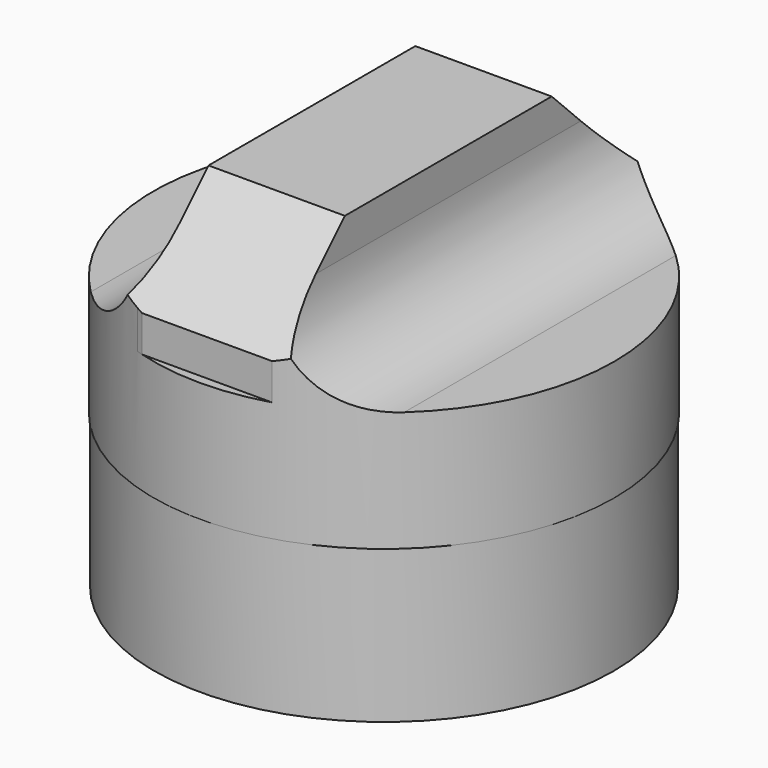
from build123d import *

# Parameters (mm, degrees)
F0_R         = 12.625
F0_R_2       = 10.375
F0_R_3       = 5
F1_DEPTH     = 15
F2_DEPTH     = 15
F3_R         = 12.6739646699
F4_DEPTH     = 6.6
F6_DEPTH     = 7
F7_T4_DEPTH  = 36.6039255786
F7_S5_R      = 12.6739646699
F7_T6_DEPTH  = 20
F7_T10_DEPTH = 24.210816556
F7_S11_R     = 12.6739646699
F7_T12_DEPTH = 14
F8_T1_DEPTH  = 32.8699146781
F9_T1_DEPTH  = 33.2150521969
F10_SCALE    = 0.79


# Not quite as in the source:
# - a fillet or chamfer that OpenCascade refuses, or shapes differently, is made with other operations: its cross-section is extruded or revolved along the edge and cut away or added
# - a feature names something its author has since deleted; it is built from what else it names


with BuildPart() as f1:
    # F0 (on Top) → F1 (new body)
    with BuildSketch(Plane.XY):
        Circle(F0_R)
        Circle(F0_R_2, mode=Mode.SUBTRACT)
        Circle(F0_R_2)
        Circle(F0_R_3, mode=Mode.SUBTRACT)
    extrude(amount=F1_DEPTH)

    # F0 (on Top) → F2 (join)
    with BuildSketch(Plane.XY):
        Circle(F0_R_3)
        with BuildLine():
            ThreePointArc((2.304625, 2.1105280404), (2.9126944678, 1.1321819366), (3.125, 0))
            ThreePointArc((3.125, 0), (-1.1321819366, -2.9126944678), (-2.304625, 2.1105280404))
            ThreePointArc((-2.304625, 2.1105280404), (0, 3.125), (2.304625, 2.1105280404))
        make_face(mode=Mode.SUBTRACT)
        with BuildLine():
            Line((-2.304625, 2.1105280404), (2.304625, 2.1105280404))
            ThreePointArc((2.304625, 2.1105280404), (0, 3.125), (-2.304625, 2.1105280404))
        make_face()
    extrude(amount=F2_DEPTH)

    # F3 (on face) → F4 (join)
    with BuildSketch(Plane.XY.offset(15)):
        Circle(F3_R)
    extrude(amount=-F4_DEPTH)

    # F5 (on face) → F6 (join)
    with BuildSketch(Plane.XY.offset(15)):
        with BuildLine():
            Line((3.5765423992, 12.0519627893), (-3.921679918, 12.0519627893))
            Line((-3.921679918, 12.0519627893), (-3.921679918, -12.0519627893))
            ThreePointArc((-3.921679918, -12.0519627893), (-3.7494920856, -12.1066382433), (-3.5765423992, -12.1588537667))
            Line((-3.5765423992, -12.1588537667), (3.5765423992, -12.1588537667))
            Line((3.5765423992, -12.1588537667), (3.5765423992, 12.0519627893))
        make_face()
    extrude(amount=F6_DEPTH)

    # F7: fillet of radius 5 on 2 edges, made by hand


with BuildPart() as f7_tool2:
    # F7_s3 → F7_t4 (new body)
    with BuildSketch(Plane.XZ.offset(-12.0519627893)):
        with BuildLine():
            ThreePointArc((-8.921679918, 15), (-5.3861460121, 16.4644660941), (-3.921679918, 20))
            Line((-3.921679918, 20), (-3.921679918, 15))
            Line((-3.921679918, 15), (-8.921679918, 15))
        make_face()
    extrude(amount=F7_T4_DEPTH)

    # F7_s5 → F7_t6 (intersect, symmetric)
    with BuildSketch(Plane.XY.offset(17.5)):
        Circle(F7_S5_R)
    extrude(amount=F7_T6_DEPTH, both=True, mode=Mode.INTERSECT)


with BuildPart() as f1_1:
    add(f1.part)

    # F7_t1: union F7_tool2
    add(f7_tool2.part)


with BuildPart() as f7_tool8:
    # F7_s9 → F7_t10 (new body)
    with BuildSketch(Plane.XZ.offset(12.1588537667)):
        with BuildLine():
            ThreePointArc((8.5765423992, 15), (5.0410084933, 16.4644660941), (3.5765423992, 20))
            Line((3.5765423992, 20), (3.5765423992, 15))
            Line((3.5765423992, 15), (8.5765423992, 15))
        make_face()
    extrude(amount=-F7_T10_DEPTH)

    # F7_s11 → F7_t12 (intersect, symmetric)
    with BuildSketch(Plane.XY.offset(17.5)):
        Circle(F7_S11_R)
    extrude(amount=F7_T12_DEPTH, both=True, mode=Mode.INTERSECT)


with BuildPart() as f1_2:
    add(f1_1.part)

    # F7_t7: union F7_tool8
    add(f7_tool8.part)

    # F8: chamfer of 5 on 1 edges, made by hand

    # F8_s2 → F8_t1 (cut)
    with BuildSketch(Plane.YZ.offset(-16.434957339)):
        Polygon((-12.1588537667, 17), (-7.1588537667, 22), (-12.1588537667, 22), align=None)
    extrude(amount=F8_T1_DEPTH, mode=Mode.SUBTRACT)

    # F9: chamfer of 5 on 1 edges, made by hand

    # F9_s2 → F9_t1 (cut)
    with BuildSketch(Plane.YZ.offset(-16.7800948578)):
        Polygon((12.0519627893, 17), (7.0519627893, 22), (12.0519627893, 22), align=None)
    extrude(amount=F9_T1_DEPTH, mode=Mode.SUBTRACT)


with BuildPart() as f1_3:
    # F10: moved
    add(f1_2.part.scale(F10_SCALE))


solid = f1_3.part
